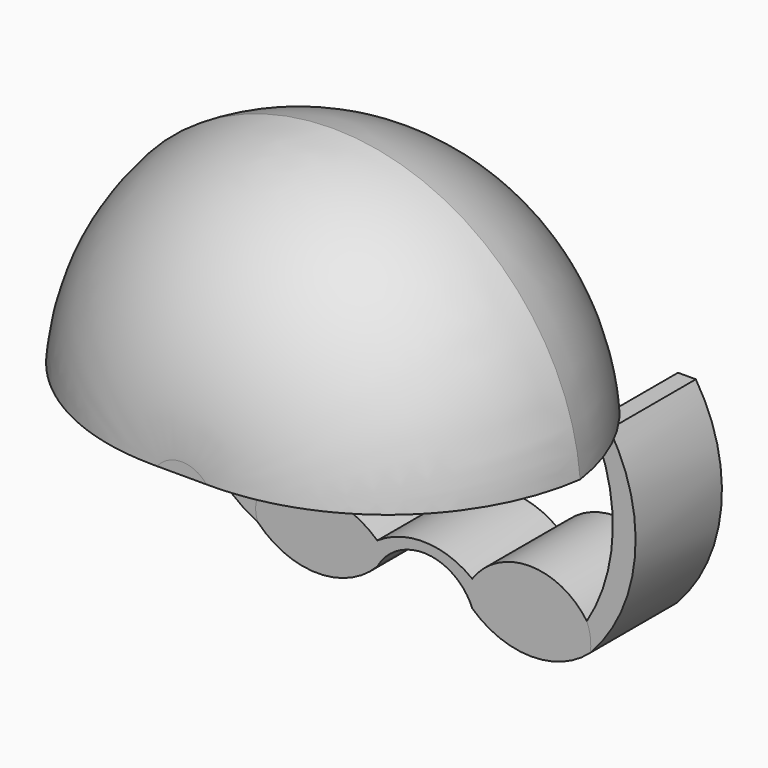
from build123d import *

# Parameters (mm, degrees)
F1_DEPTH    = 88.9
F2_T2_ANGLE = 359.64
F2_T4_ANGLE = 359.64
F4_DEPTH    = 25.4
F5_DEPTH    = 25.4


# Not quite as in the source:
# - a fillet or chamfer that OpenCascade refuses, or shapes differently, is made with other operations: its cross-section is extruded or revolved along the edge and cut away or added


with BuildPart() as f1:
    # F0 (on Front) → F1 (new body)
    with BuildSketch(Plane.XZ):
        with BuildLine():
            ThreePointArc((59.5757886767, 19.8585987091), (0.8634161204, 74.170312897), (-57.8489564359, 19.8585987091))
            Line((-57.8489564359, 19.8585987091), (59.5757886767, 19.8585987091))
        make_face()
    extrude(amount=F1_DEPTH)

    # F2: fillet of radius 51.5096605668 on 2 edges, made by hand

    # F2_s1 → F2_t2 (revolve, cut)
    with BuildSketch(Plane(origin=(0.9114097399, 0, 0.0028632876), x_dir=(0, 1, 0), z_dir=(-0.9999950652, 0, -0.0031415875))):
        with BuildLine():
            ThreePointArc((-37.3903394332, 43.6137876504), (-73.8131697166, 28.526957367), (-88.9, -7.8958729164))
            Line((-88.9, -7.8958729164), (-88.9, 43.6137876504))
            Line((-88.9, 43.6137876504), (-37.3903394332, 43.6137876504))
        make_face()
    revolve(axis=Axis((0.8634161204, -88.9, 15.2796565729), (0, -1, 0)), revolution_arc=F2_T2_ANGLE, mode=Mode.SUBTRACT)

    # F2_s3 → F2_t4 (revolve, cut)
    with BuildSketch(Plane(origin=(0.9114097399, 0, 0.0028632876), x_dir=(0, 1, 0), z_dir=(-0.9999950652, 0, -0.0031415875))):
        with BuildLine():
            ThreePointArc((-51.5096605668, 43.6137876504), (-15.0868302834, 28.526957367), (0, -7.8958729164))
            Line((0, -7.8958729164), (0, 43.6137876504))
            Line((0, 43.6137876504), (-51.5096605668, 43.6137876504))
        make_face()
    revolve(axis=Axis((0.8634161204, 0, 15.2796565729), (0, -1, 0)), revolution_arc=F2_T4_ANGLE, mode=Mode.SUBTRACT)


with BuildPart() as f4:
    # F3 (on Front) → F4 (new body)
    with BuildSketch(Plane.XZ):
        with BuildLine():
            ThreePointArc((-31.9720953703, -21.0119523108), (-32.5286170117, -23.7042130902), (-31.9720953703, -26.3964738697))
            ThreePointArc((-31.9720953703, -26.3964738697), (-17.9338779999, -32.3648560237), (-3.8956606295, -26.3964738697))
            ThreePointArc((-3.8956606295, -26.3964738697), (-3.7989683826, -26.2248697788), (-3.6995589857, -26.0548252952))
            ThreePointArc((-3.6995589857, -26.0548252952), (-3.1254057527, -23.5072488783), (-3.8956606295, -21.0119523108))
            ThreePointArc((-3.8956606295, -21.0119523108), (-17.9338779999, -15.5918990312), (-31.9720953703, -21.0119523108))
        make_face()
        with BuildLine():
            ThreePointArc((18.44827272, -21.6751024127), (17.3677793216, -23.437783574), (17.2320588287, -25.5008130959))
            ThreePointArc((17.2320588287, -25.5008130959), (17.9013139449, -26.6247801583), (18.44827272, -27.8130732477))
            ThreePointArc((18.44827272, -27.8130732477), (32.308258524, -33.2615091406), (46.2306588888, -27.9745981097))
            ThreePointArc((46.2306588888, -27.9745981097), (46.2561820848, -24.7698070026), (45.4230308533, -21.6751024127))
            ThreePointArc((45.4230308533, -21.6751024127), (31.9356517866, -14.6190424345), (18.44827272, -21.6751024127))
        make_face()
        with BuildLine():
            ThreePointArc((-3.8956606295, -21.0119523108), (-3.1254057527, -23.5072488783), (-3.6995589857, -26.0548252952))
            ThreePointArc((-3.6995589857, -26.0548252952), (6.6135950932, -20.0102340616), (17.2320588287, -25.5008130959))
            ThreePointArc((17.2320588287, -25.5008130959), (17.3677793216, -23.437783574), (18.44827272, -21.6751024127))
            ThreePointArc((18.44827272, -21.6751024127), (7.383863358, -17.7195311955), (-3.8956606295, -21.0119523108))
        make_face()
    extrude(amount=F4_DEPTH)


with BuildPart() as f5:
    # F3 (on Front) → F5 (new body)
    with BuildSketch(Plane.XZ):
        with BuildLine():
            Line((-43.8949614763, 19.8847707361), (-49.4076870382, 19.8037457436))
            ThreePointArc((-49.4076870382, 19.8037457436), (-49.694155963, -6.6945012346), (-31.9720953703, -26.3964738697))
            ThreePointArc((-31.9720953703, -26.3964738697), (-32.5286170117, -23.7042130902), (-31.9720953703, -21.0119523108))
            ThreePointArc((-31.9720953703, -21.0119523108), (-45.6760319405, -2.820809114), (-43.8949614763, 19.8847707361))
        make_face()
    extrude(amount=F5_DEPTH)


with BuildPart() as f5b:
    # F3 (on Front) → F5, piece 2 (new body)
    with BuildSketch(Plane.XZ):
        with BuildLine():
            ThreePointArc((46.5537086129, 19.8369566351), (51.5130220007, -1.0695496802), (45.4230308533, -21.6751024127))
            ThreePointArc((45.4230308533, -21.6751024127), (46.2561820848, -24.7698070026), (46.2306588888, -27.9745981097))
            ThreePointArc((46.2306588888, -27.9745981097), (56.7231845264, -4.8474447832), (50.7533736527, 19.8369566351))
            Line((50.7533736527, 19.8369566351), (46.5537086129, 19.8369566351))
        make_face()
    extrude(amount=F5_DEPTH)


solid = Compound([f1.part, f4.part, f5.part, f5b.part])
